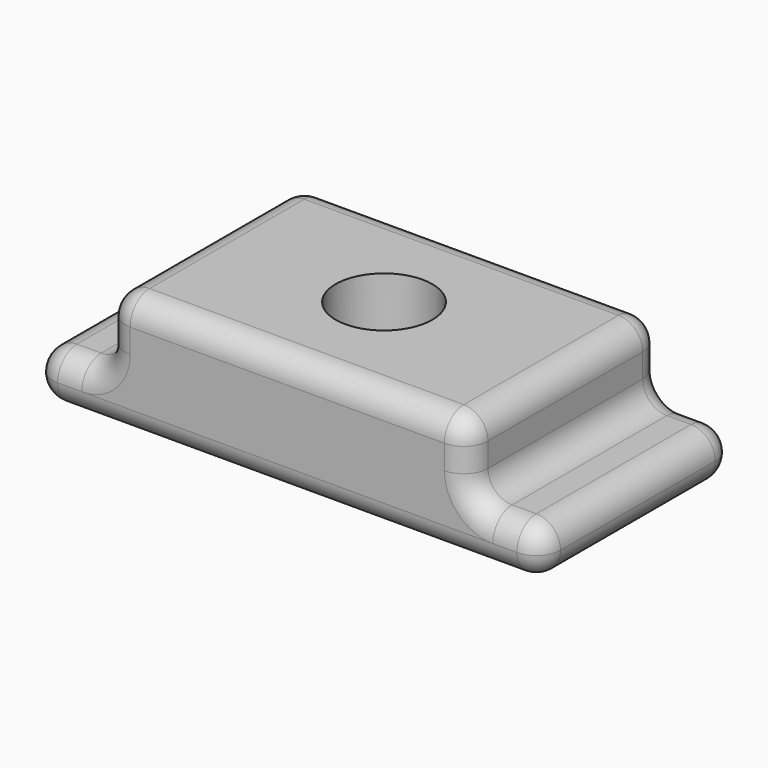
from build123d import *

# Parameters (mm, degrees)
F0_W     = 15
F0_H     = 10
F0_R     = 3.5
F1_DEPTH = 5
F0_W_2   = 3
F2_DEPTH = 2
F3_R     = 0.99999
F0_R_2   = 2
F4_DEPTH = 5
F5_SIZE  = 1.5


# Not quite as in the source:
# - a fillet or chamfer is up to 0.001 mm smaller than in the source, because OpenCascade refuses the exact size


with BuildPart() as f1:
    # F0 (on Top) → F1 (new body)
    with BuildSketch(Plane.XY):
        with Locations((7.5, -5)):
            Rectangle(F0_W, F0_H)
        with Locations((7.5, -5)):
            Circle(F0_R, mode=Mode.SUBTRACT)
    extrude(amount=F1_DEPTH)

    # F0 (on Top) → F2 (join)
    with BuildSketch(Plane.XY):
        with Locations((-1.5, -5)):
            Rectangle(F0_W_2, F0_H)
        with Locations((16.5, -5)):
            Rectangle(F0_W_2, F0_H)
    extrude(amount=F2_DEPTH)

    # F3 (radius 1 in the source; OpenCascade refuses exactly that, so slightly less here)
    f3_edges = [f1.edges().sort_by_distance(p)[0] for p in [
        (15, 0, 3.5),
        (7.5, 0, 5),
        (0, 0, 3.5),
        (-1.5, 0, 2),
        (-3, 0, 1),
        (7.5, 0, 0),
        (18, 0, 1),
        (16.5, 0, 2),
        (0, -10, 3.5),
        (7.5, -10, 5),
        (15, -10, 3.5),
        (16.5, -10, 2),
        (18, -10, 1),
        (7.5, -10, 0),
        (-3, -10, 1),
        (-1.5, -10, 2),
        (15, -5, 2),
        (15, -5, 5),
        (18, -5, 0),
        (18, -5, 2),
        (0, -5, 2),
        (-3, -5, 2),
        (0, -5, 5),
        (-3, -5, 0),
    ]]
    fillet(f3_edges, radius=F3_R)

    # F0 (on Top) → F4 (join)
    with BuildSketch(Plane.XY):
        with Locations((7.5, -5)):
            Circle(F0_R)
        with Locations((7.5, -5)):
            Circle(F0_R_2, mode=Mode.SUBTRACT)
    extrude(amount=F4_DEPTH)

    # F5
    f5_edges = [f1.edges().sort_by_distance(p)[0] for p in [
        (5.5, -5, 0),
    ]]
    chamfer(f5_edges, length=F5_SIZE)


solid = f1.part
